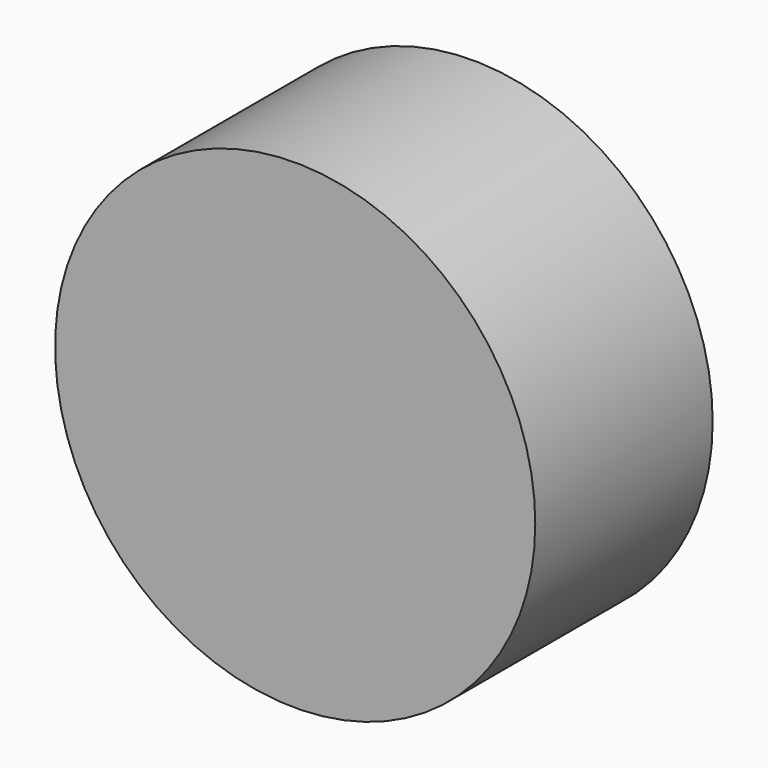
from build123d import *

# Parameters (mm, degrees)
F0_R         = 27.5
F0_R_2       = 20.5
F0_R_3       = 3.3756193286
F0_R_4       = 3.1618602981
F0_R_5       = 4
F0_TEXT_SIZE = 17.1353199726
F1_DEPTH     = 25.4


# Not quite as in the source:
# - Text() gives the source's letters only with a copy of the font that has no kerning and outlines rounded to 1/6400 em; it was checked with that copy


with BuildPart() as f1:
    # F0 (on Front) → F1 (new body)
    with BuildSketch(Plane.XZ):
        with Locations((-4.6842060983, 10.8692832291)):
            Circle(F0_R)
        with Locations((-4.6842060983, 10.8692832291)):
            Circle(F0_R_2, mode=Mode.SUBTRACT)
        with Locations((-4.6842060983, 10.8692832291)):
            Circle(F0_R_2)
        Polygon((-2.2001986314, 3.4657486249), (-4.995397702, 3.4657486249), (-5.8816150318, 6.3787530202), (-10.3421530122, 6.3787530202), (-11.228370342, 3.4657486249), (-14.0235694125, 3.4657486249), (-9.7049333007, 15.7496311302), (-6.5348991057, 15.7496311302), align=None, mode=Mode.SUBTRACT)
        with BuildLine():
            add(Edge.make_bspline(
                [(5.8989174494, 13.4725077495), (5.2054724692, 13.7148118835), (4.5361240328, 13.7148118835)],
                knots=[0, 0, 0, 1, 1, 1], degree=2))
            add(Edge.make_bspline(
                [(4.5361240328, 13.7148118835), (3.0715896539, 13.7148118835), (2.2683715302, 12.614403054)],
                knots=[0, 0, 0, 1, 1, 1], degree=2))
            add(Edge.make_bspline(
                [(2.2683715302, 12.614403054), (1.4651534065, 11.5139942245), (1.4651534065, 9.5487872152)],
                knots=[0, 0, 0, 1, 1, 1], degree=2))
            add(Edge.make_bspline(
                [(1.4651534065, 9.5487872152), (1.4651534065, 5.4577295717), (4.5361240328, 5.4577295717)],
                knots=[0, 0, 0, 1, 1, 1], degree=2))
            add(Edge.make_bspline(
                [(4.5361240328, 5.4577295717), (5.8239504245, 5.4577295717), (7.6552877466, 6.1003040707)],
                knots=[0, 0, 0, 1, 1, 1], degree=2))
            Line((7.6552877466, 6.1003040707), (7.6552877466, 3.9262603491))
            add(Edge.make_bspline(
                [(7.6552877466, 3.9262603491), (6.1505924615, 3.2970728189), (4.292481202, 3.2970728189)],
                knots=[0, 0, 0, 1, 1, 1], degree=2))
            add(Edge.make_bspline(
                [(4.292481202, 3.2970728189), (1.6231196375, 3.2970728189), (0.2094557397, 4.9168960351)],
                knots=[0, 0, 0, 1, 1, 1], degree=2))
            add(Edge.make_bspline(
                [(0.2094557397, 4.9168960351), (-1.204208158, 6.5367192512), (-1.204208158, 9.5648515776)],
                knots=[0, 0, 0, 1, 1, 1], degree=2))
            add(Edge.make_bspline(
                [(-1.204208158, 9.5648515776), (-1.204208158, 11.4738333183), (-0.509424481, 12.908916366)],
                knots=[0, 0, 0, 1, 1, 1], degree=2))
            add(Edge.make_bspline(
                [(-0.509424481, 12.908916366), (0.185359196, 14.3439994137), (1.4865725564, 15.1083953281)],
                knots=[0, 0, 0, 1, 1, 1], degree=2))
            add(Edge.make_bspline(
                [(1.4865725564, 15.1083953281), (2.7877859169, 15.8727912425), (4.5361240328, 15.8727912425)],
                knots=[0, 0, 0, 1, 1, 1], degree=2))
            add(Edge.make_bspline(
                [(4.5361240328, 15.8727912425), (6.3165908737, 15.8727912425), (8.1157994708, 15.0133478502)],
                knots=[0, 0, 0, 1, 1, 1], degree=2))
            Line((8.1157994708, 15.0133478502), (7.2804526222, 12.9035615785))
            add(Edge.make_bspline(
                [(7.2804526222, 12.9035615785), (6.5923624295, 13.2302036155), (5.8989174494, 13.4725077495)],
                knots=[0, 0, 0, 1, 1, 1], degree=2))
        make_face(mode=Mode.SUBTRACT)
        with Locations((-18.5727346689, 10.8692832291)):
            Circle(F0_R_3, mode=Mode.SUBTRACT)
        with Locations((-4.9861297011, 25.9655099362)):
            Circle(F0_R_4, mode=Mode.SUBTRACT)
        with Locations((6.222014246, 21.2711636585)):
            Circle(F0_R_5, mode=Mode.SUBTRACT)
        with Locations((-14.0235694125, 3.4657486249)):
            Text('AC', F0_TEXT_SIZE, font='Open Sans', font_style=FontStyle.BOLD, text_align=(TextAlign.LEFT, TextAlign.BOTTOM))
        with Locations((6.222014246, 21.2711636585)):
            Circle(F0_R_5)
        with Locations((-18.5727346689, 10.8692832291)):
            Circle(F0_R_3)
        with Locations((-4.9861297011, 25.9655099362)):
            Circle(F0_R_4)
        with BuildLine():
            Line((-9.6888689382, 8.5527967417), (-6.5027703808, 8.5527967417))
            add(Edge.make_bspline(
                [(-6.5027703808, 8.5527967417), (-7.7316941101, 12.5099846979), (-7.8869829473, 13.0293990846)],
                knots=[0, 0, 0, 1, 1, 1], degree=2))
            add(Edge.make_bspline(
                [(-7.8869829473, 13.0293990846), (-8.0422717846, 13.5488134713), (-8.1092066282, 13.8486815708)],
                knots=[0, 0, 0, 1, 1, 1], degree=2))
            add(Edge.make_bspline(
                [(-8.1092066282, 13.8486815708), (-8.384978184, 12.7777240725), (-9.6888689382, 8.5527967417)],
                knots=[0, 0, 0, 1, 1, 1], degree=2))
        make_face()
    extrude(amount=F1_DEPTH)


solid = f1.part
